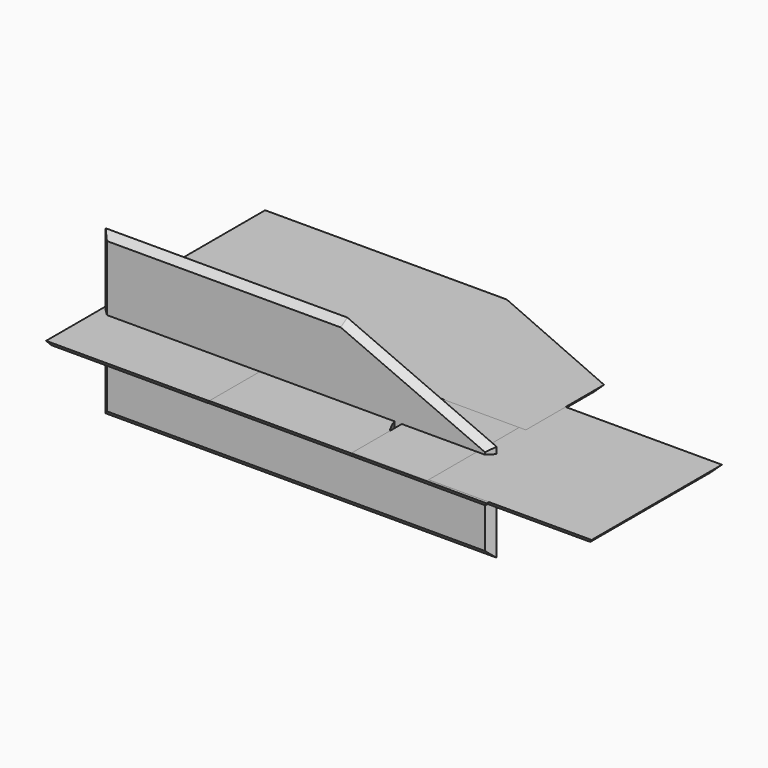
from build123d import *

# Parameters (mm, degrees)
F0_W      = 120
F0_H      = 50
F0_R      = 10.6084843686
F0_R_2    = 20
F1_DEPTH  = 2
F2_W      = 50
F2_H      = 50
F3_DEPTH  = 2
F4_W      = 30
F4_H      = 50
F5_DEPTH  = 2
F6_W      = 50
F6_H      = 50
F7_DEPTH  = 2
F9_DEPTH  = 2
F11_DEPTH = 2
F12_SIZE  = 1.99999
F13_SIZE  = 1.99999
F14_SIZE  = 1.99999
F15_SIZE  = 1.99999
F16_SIZE  = 1.99999
F17_SIZE  = 1.99999


# Not quite as in the source:
# - a fillet or chamfer is up to 0.001 mm smaller than in the source, because OpenCascade refuses the exact size


with BuildPart() as f1:
    # F0 (on Top) → F1 (new body)
    with BuildSketch(Plane.XY):
        with Locations((11.2693273971, 3.541611135)):
            Rectangle(F0_W, F0_H)
        with Locations((-23.7306726029, 4.672499537)):
            Circle(F0_R, mode=Mode.SUBTRACT)
        with Locations((46.2693273971, 4.5276646413)):
            Circle(F0_R_2, mode=Mode.SUBTRACT)
    extrude(amount=F1_DEPTH)

    # F12 (size 2 in the source; OpenCascade refuses exactly that, so slightly less here)
    f12_edges = [f1.edges().sort_by_distance(p)[0] for p in [
        (71.269327, 3.541611, 0),
        (11.269327, 28.541611, 0),
        (-48.730673, 3.541611, 0),
        (11.269327, -21.458389, 0),
    ]]
    chamfer(f12_edges, length=F12_SIZE)


with BuildPart() as f3:
    # F2 (on Top) → F3 (new body)
    with BuildSketch(Plane.XY):
        with Locations((-38.8736227571, 3.468115814)):
            Rectangle(F2_W, F2_H)
    extrude(amount=F3_DEPTH)

    # F13 (size 2 in the source; OpenCascade refuses exactly that, so slightly less here)
    f13_edges = [f3.edges().sort_by_distance(p)[0] for p in [
        (-38.873623, -21.531884, 0),
        (-13.873623, 3.468116, 0),
        (-38.873623, 28.468116, 0),
    ]]
    chamfer(f13_edges, length=F13_SIZE)


with BuildPart() as f5:
    # F4 (on Top) → F5 (new body)
    with BuildSketch(Plane.XY):
        with Locations((44.6629953704, 3.9126975462)):
            Rectangle(F4_W, F4_H)
    extrude(amount=F5_DEPTH)

    # F14 (size 2 in the source; OpenCascade refuses exactly that, so slightly less here)
    f14_edges = [f5.edges().sort_by_distance(p)[0] for p in [
        (44.662995, -21.087302, 0),
        (29.662995, 3.912698, 0),
        (44.662995, 28.912698, 0),
        (59.662995, 3.912698, 0),
    ]]
    chamfer(f14_edges, length=F14_SIZE)


with BuildPart() as f7:
    # F6 (on Top) → F7 (new body)
    with BuildSketch(Plane.XY):
        with Locations((77.7432139613, 4.4250842184)):
            Rectangle(F6_W, F6_H)
    extrude(amount=F7_DEPTH)

    # F15 (size 2 in the source; OpenCascade refuses exactly that, so slightly less here)
    f15_edges = [f7.edges().sort_by_distance(p)[0] for p in [
        (77.743214, -20.574916, 0),
        (52.743214, 4.425084, 0),
        (77.743214, 29.425084, 0),
        (102.743214, 4.425084, 0),
    ]]
    chamfer(f15_edges, length=F15_SIZE)


with BuildPart() as f9:
    # F8 (on Top) → F9 (new body)
    with BuildSketch(Plane.XY):
        Polygon((-65.216818493, 64.1614470469), (-65.216818493, 14.1614470469), (54.783181507, 14.1614470469), (54.783181507, 44.1614470469), (8.9574245575, 64.1614470469), align=None)
    extrude(amount=F9_DEPTH)

    # F16 (size 2 in the source; OpenCascade refuses exactly that, so slightly less here)
    f16_edges = [f9.edges().sort_by_distance(p)[0] for p in [
        (-5.216818, 14.161447, 0),
        (-65.216818, 39.161447, 0),
        (54.783182, 29.161447, 0),
        (31.870303, 54.161447, 0),
    ]]
    chamfer(f16_edges, length=F16_SIZE)


with BuildPart() as f11:
    # F10 (on Front) → F11 (new body)
    with BuildSketch(Plane.XZ):
        Polygon((-62.8348486101, 24), (-62.8348486101, -26), (57.1651513899, -26), (57.1651513899, 4), (11.3393944404, 24), align=None)
    extrude(amount=F11_DEPTH)

    # F17 (size 2 in the source; OpenCascade refuses exactly that, so slightly less here)
    f17_edges = [f11.edges().sort_by_distance(p)[0] for p in [
        (34.252273, -2, 14),
        (-25.747727, -2, 24),
        (-62.834849, -2, -1),
        (57.165151, -2, -11),
        (-2.834849, -2, -26),
    ]]
    chamfer(f17_edges, length=F17_SIZE)


solid = Compound([f1.part, f3.part, f5.part, f7.part, f9.part, f11.part])
